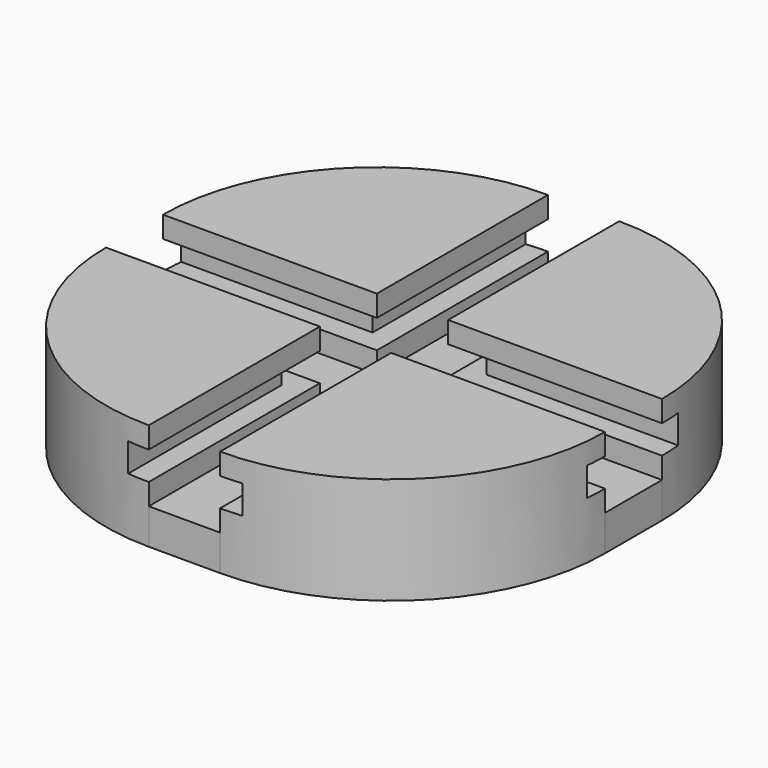
from build123d import *

# Parameters (mm, degrees)
F0_W        = 88.9
F0_H        = 88.9
F1_DEPTH    = 19.05
F3_DEPTH    = 12.7
F4_T1_DEPTH = 209.55
F5_W        = 3.81
F5_H        = 5.08
F6_DEPTH    = 38.1
F7_W        = 3.81
F7_H        = 5.08
F8_DEPTH    = 38.1
F9_W        = 3.81
F9_H        = 5.08
F10_DEPTH   = 38.1
F11_W       = 3.81
F11_H       = 5.08
F12_DEPTH   = 38.1
F13_W       = 3.81
F13_H       = 5.08
F14_DEPTH   = 38.1
F15_W       = 3.81
F15_H       = 5.08
F16_DEPTH   = 38.1
F17_W       = 3.81
F17_H       = 5.08
F18_DEPTH   = 38.1
F19_W       = 3.81
F19_H       = 5.08
F20_DEPTH   = 38.1


# Not quite as in the source:
# - a fillet or chamfer that OpenCascade refuses, or shapes differently, is made with other operations: its cross-section is extruded or revolved along the edge and cut away or added


with BuildPart() as f1:
    # F0 (on Top) → F1 (new body)
    with BuildSketch(Plane.XY):
        with Locations((44.45, 44.45)):
            Rectangle(F0_W, F0_H)
    extrude(amount=F1_DEPTH)

    # F2 (on face) → F3 (cut)
    with BuildSketch(Plane.XY.offset(19.05)):
        Polygon((38.1, 50.8), (0, 50.8), (0, 38.1), (38.1, 38.1), (38.1, 0), (50.8, 0), (50.8, 38.1), (88.9, 38.1), (88.9, 50.8), (50.8, 50.8), (50.8, 88.9), (38.1, 88.9), align=None)
    extrude(amount=-F3_DEPTH, mode=Mode.SUBTRACT)

    # F4: fillet of radius 38.1 on 4 edges, made by hand

    # F4_s2 → F4_t1 (cut)
    with BuildSketch(Plane.XY.offset(-95.25)):
        with BuildLine():
            ThreePointArc((50.8, 0), (77.7407683632, 11.1592316368), (88.9, 38.1))
            Line((88.9, 38.1), (88.9, 0))
            Line((88.9, 0), (50.8, 0))
        make_face()
        with BuildLine():
            ThreePointArc((0, 38.1), (11.1592316368, 11.1592316368), (38.1, 0))
            Line((38.1, 0), (0, 0))
            Line((0, 0), (0, 38.1))
        make_face()
        with BuildLine():
            ThreePointArc((50.8, 88.9), (77.7407683632, 77.7407683632), (88.9, 50.8))
            Line((88.9, 50.8), (88.9, 88.9))
            Line((88.9, 88.9), (50.8, 88.9))
        make_face()
        with BuildLine():
            ThreePointArc((0, 50.8), (11.1592316368, 77.7407683632), (38.1, 88.9))
            Line((38.1, 88.9), (0, 88.9))
            Line((0, 88.9), (0, 50.8))
        make_face()
    extrude(amount=F4_T1_DEPTH, mode=Mode.SUBTRACT)

    # F5 (on face) → F6 (cut)
    with BuildSketch(Plane(origin=(0, 38.1, 0), x_dir=(-1, 0, 0), z_dir=(0, 1, 0))):
        with Locations((-52.705, 12.7)):
            Rectangle(F5_W, F5_H)
    extrude(amount=-F6_DEPTH, mode=Mode.SUBTRACT)

    # F7 (on face) → F8 (cut)
    with BuildSketch(Plane.XZ.offset(-50.8)):
        with Locations((52.705, 12.7)):
            Rectangle(F7_W, F7_H)
    extrude(amount=-F8_DEPTH, mode=Mode.SUBTRACT)

    # F9 (on face) → F10 (cut)
    with BuildSketch(Plane.YZ.offset(38.1)):
        with Locations((36.195, 12.7)):
            Rectangle(F9_W, F9_H)
    extrude(amount=-F10_DEPTH, mode=Mode.SUBTRACT)

    # F11 (on face) → F12 (cut)
    with BuildSketch(Plane(origin=(54.61, 0, 0), x_dir=(0, -1, 0), z_dir=(-1, 0, 0))):
        with Locations((-36.195, 12.7)):
            Rectangle(F11_W, F11_H)
    extrude(amount=-F12_DEPTH, mode=Mode.SUBTRACT)

    # F13 (on face) → F14 (cut)
    with BuildSketch(Plane.YZ.offset(38.1)):
        with Locations((52.705, 12.7)):
            Rectangle(F13_W, F13_H)
    extrude(amount=-F14_DEPTH, mode=Mode.SUBTRACT)

    # F15 (on face) → F16 (cut)
    with BuildSketch(Plane(origin=(54.61, 0, 0), x_dir=(0, -1, 0), z_dir=(-1, 0, 0))):
        with Locations((-52.705, 12.7)):
            Rectangle(F15_W, F15_H)
    extrude(amount=-F16_DEPTH, mode=Mode.SUBTRACT)

    # F17 (on face) → F18 (cut)
    with BuildSketch(Plane.XZ.offset(-54.61)):
        with Locations((36.195, 12.7)):
            Rectangle(F17_W, F17_H)
    extrude(amount=-F18_DEPTH, mode=Mode.SUBTRACT)

    # F19 (on face) → F20 (cut)
    with BuildSketch(Plane(origin=(0, 34.29, 0), x_dir=(-1, 0, 0), z_dir=(0, 1, 0))):
        with Locations((-36.195, 12.7)):
            Rectangle(F19_W, F19_H)
    extrude(amount=-F20_DEPTH, mode=Mode.SUBTRACT)


solid = f1.part
